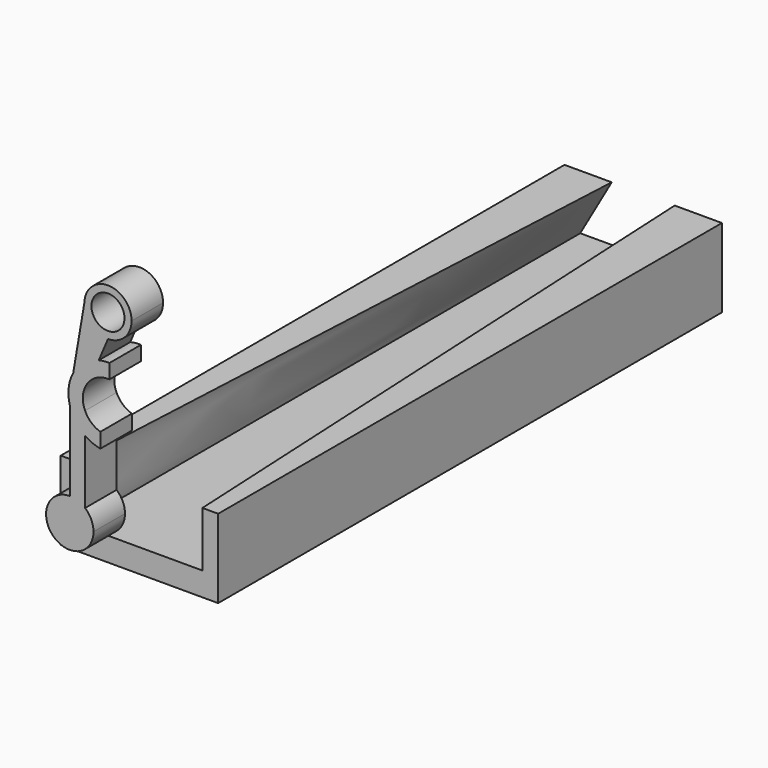
from build123d import *

# Parameters (mm, degrees)
F0_W     = 20
F0_H     = 10
F1_DEPTH = 80
F2_W     = 16
F2_H     = 7
F5_R     = 2.1
F6_DEPTH = 5


with BuildPart() as f1:
    # F0 (on Front) → F1 (new body)
    with BuildSketch(Plane.XZ):
        with Locations((0, 5)):
            Rectangle(F0_W, F0_H)
    extrude(amount=-F1_DEPTH)

    # F2 (on face) → F4 section 0
    with BuildSketch(Plane.XZ):
        with Locations((0, 6.5)):
            Rectangle(F2_W, F2_H)
    # F3 (on face) → F4 section 1
    with BuildSketch(Plane(origin=(0, 80, 0), x_dir=(-1, 0, 0), z_dir=(0, 1, 0))):
        Polygon((4, 10), (-4, 10), (-8, 3), (8, 3), align=None)
    loft(mode=Mode.SUBTRACT)


with BuildPart() as f6:
    # F5 (on Front) → F6 (new body)
    with BuildSketch(Plane.XZ):
        with BuildLine():
            Line((-4.8518124968, 6.1728735454), (-4.8518124968, 9.1862847298))
            ThreePointArc((-4.8518124968, 9.1862847298), (-6.9826159798, 4.0420700624), (-1.8384013124, 6.1728735454))
            ThreePointArc((-1.8384013124, 6.1728735454), (-2.118757562, 7.4421480192), (-2.9076597649, 8.4752456095))
            Line((-2.9076597649, 8.4752456095), (-2.9076597649, 6.1728735454))
            Line((-2.9076597649, 6.1728735454), (-4.8518124968, 6.1728735454))
        make_face()
        with BuildLine():
            ThreePointArc((-2.9076597649, 8.4752456095), (-3.8167634067, 9.0029478108), (-4.8518124968, 9.1862847298))
            Line((-4.8518124968, 9.1862847298), (-4.8518124968, 6.1728735454))
            Line((-4.8518124968, 6.1728735454), (-2.9076597649, 6.1728735454))
            Line((-2.9076597649, 6.1728735454), (-2.9076597649, 8.4752456095))
        make_face()
        with BuildLine():
            ThreePointArc((-2.9076597649, 16.5737187745), (-4.1210807971, 17.7944757075), (-4.8518124968, 19.3528945454))
            Line((-4.8518124968, 19.3528945454), (-4.8518124968, 9.1862847298))
            ThreePointArc((-4.8518124968, 9.1862847298), (-3.8167634067, 9.0029478108), (-2.9076597649, 8.4752456095))
            Line((-2.9076597649, 8.4752456095), (-2.9076597649, 16.5737187745))
        make_face()
        with BuildLine():
            ThreePointArc((-0.9662810217, 17.6318659056), (-2.1195139064, 18.2864649445), (-2.9076597649, 19.3528945454))
            Line((-2.9076597649, 19.3528945454), (-2.9076597649, 16.5737187745))
            ThreePointArc((-2.9076597649, 16.5737187745), (-1.9811399388, 16.0546494321), (-0.9662810217, 15.7417063883))
            Line((-0.9662810217, 15.7417063883), (-0.9662810217, 17.6318659056))
        make_face()
        with BuildLine():
            Line((-2.9076597649, 19.3528945454), (-4.8518124968, 19.3528945454))
            ThreePointArc((-4.8518124968, 19.3528945454), (-4.1210807971, 17.7944757075), (-2.9076597649, 16.5737187745))
            Line((-2.9076597649, 16.5737187745), (-2.9076597649, 19.3528945454))
        make_face()
        with BuildLine():
            ThreePointArc((-1.1679330145, 25.5691985063), (-3.0562313548, 24.6715585269), (-4.4163428976, 23.0836275632))
            ThreePointArc((-4.4163428976, 23.0836275632), (-4.9954247383, 21.2604392671), (-4.8518124968, 19.3528945454))
            Line((-4.8518124968, 19.3528945454), (-2.9076597649, 19.3528945454))
            ThreePointArc((-2.9076597649, 19.3528945454), (-2.634816389, 22.4846688372), (0.1886498126, 23.8668744407))
            Line((0.1886498126, 23.8668744407), (0.1886498126, 25.7031494596))
            ThreePointArc((0.1886498126, 25.7031494596), (-0.4942009833, 25.6823489417), (-1.1679330145, 25.5691985063))
        make_face()
        with BuildLine():
            ThreePointArc((0, 28.3258753854), (-2.1433167436, 29.2267819295), (-2.9993481003, 31.388413161))
            Line((-2.9993481003, 31.388413161), (-4.4163428976, 23.0836275632))
            ThreePointArc((-4.4163428976, 23.0836275632), (-3.0562313548, 24.6715585269), (-1.1679330145, 25.5691985063))
            Line((-1.1679330145, 25.5691985063), (0, 28.3258753854))
        make_face()
        with BuildLine():
            ThreePointArc((0, 28.3258753854), (2.1213203436, 29.2045550419), (3, 31.3258753854))
            ThreePointArc((3, 31.3258753854), (0.0312705866, 34.3257124061), (-2.9993481003, 31.388413161))
            ThreePointArc((-2.9993481003, 31.388413161), (-2.1433167436, 29.2267819295), (0, 28.3258753854))
        make_face()
        with Locations((0, 31.3258753854)):
            Circle(F5_R, mode=Mode.SUBTRACT)
    extrude(amount=F6_DEPTH)


solid = Compound([f1.part, f6.part])
